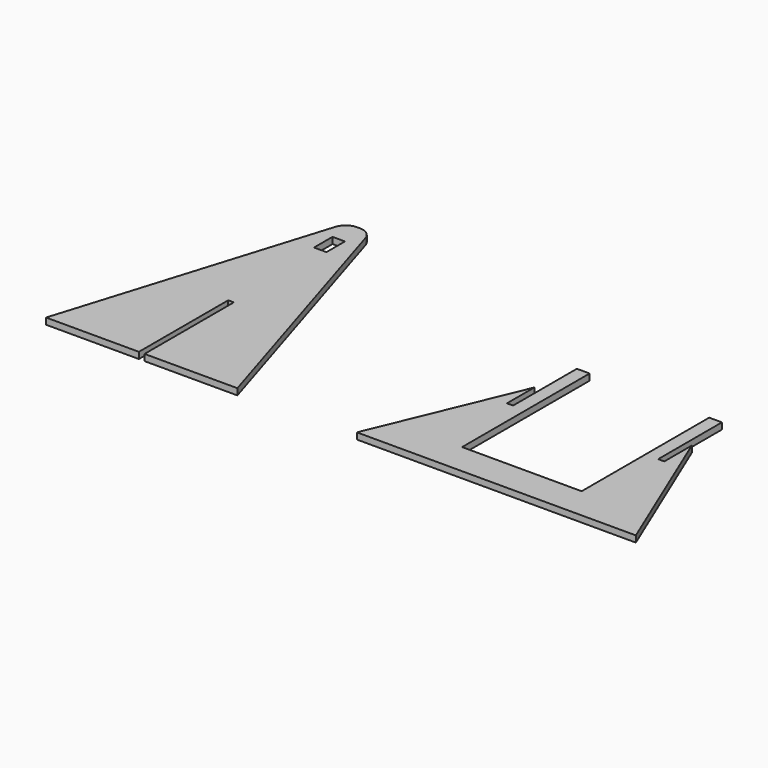
from build123d import *

# Parameters (mm, degrees)
F0_W     = 7.8
F0_H     = 14.5
F1_DEPTH = 4


# Not quite as in the source:
# - a feature names something its author has since deleted; it is built from what else it names


with BuildPart() as f1:
    # F0 (on Top) → F1 (new body)
    with BuildSketch(Plane.XY):
        with BuildLine():
            Line((-59.1399900081, 87.8836867213), (-60.8600099919, 87.8836867213))
            ThreePointArc((-60.8600099919, 87.8836867213), (-66.2031870254, 86.1259556468), (-69.4592822125, 81.5393443189))
            Line((-69.4592822125, 81.5393443189), (-120, -82.1163132787))
            Line((-120, -82.1163132787), (-61.775, -82.1163132787))
            Line((-61.775, -82.1163132787), (-61.775, -12.1163132787))
            Line((-61.775, -12.1163132787), (-58.225, -12.1163132787))
            Line((-58.225, -12.1163132787), (-58.225, -82.1163132787))
            Line((-58.225, -82.1163132787), (0, -82.1163132787))
            Line((0, -82.1163132787), (-50.5407177875, 81.5393443189))
            ThreePointArc((-50.5407177875, 81.5393443189), (-53.7968129746, 86.1259556468), (-59.1399900081, 87.8836867213))
        make_face()
        with Locations((-60, 65.1336867213)):
            Rectangle(F0_W, F0_H, mode=Mode.SUBTRACT)
    extrude(amount=F1_DEPTH)


with BuildPart() as f1b:
    # F0 (on Top) → F1, piece 2 (new body)
    with BuildSketch(Plane.XY):
        Polygon((125, -82.1163132787), (200, -82.1163132787), (250, -82.1163132787), (211.85, 9.4436867213), (211.85, -12.1163132787), (208, -12.1163132787), (208, 18.6836867213), (208, 37.8836867213), (200, 37.8836867213), (200, 24.5272498578), (200, -62.1163132787), (125, -62.1163132787), (125, 24.5272498578), (125, 37.8836867213), (117, 37.8836867213), (117, 18.6836867213), (117, -12.1163132787), (113.15, -12.1163132787), (113.15, 9.4436867213), (75, -82.1163132787), align=None)
    extrude(amount=F1_DEPTH)


solid = Compound([f1.part, f1b.part])
